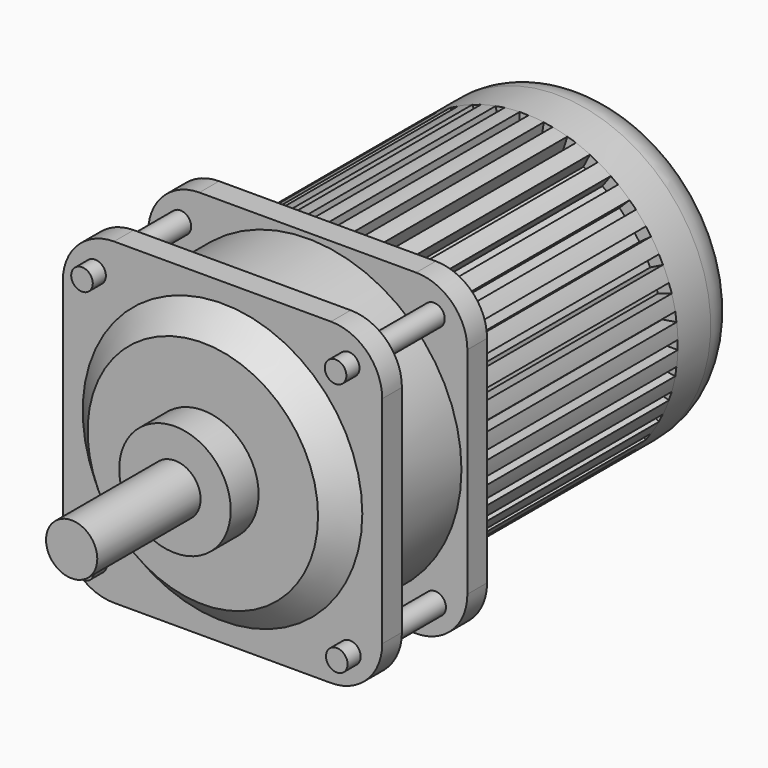
from build123d import *

# Parameters (mm, degrees)
F0_R           = 19.0502006096
F1_DEPTH       = 15.24
F1_DEPTH_BACK  = 15.24
F2_W           = 1.1123471195
F2_H           = 2.4813897908
F2_W_2         = 2.4813897908
F2_H_2         = 1.1123471195
F3_DEPTH       = 35.56
F4_R           = 19.0502006096
F5_DEPTH       = 10.16
F6_R           = 5.08
F8_DEPTH       = 3.048
F9_R           = 19.0452991295
F10_DEPTH      = 10.16
F12_DEPTH      = 3.048
F13_R          = 17.3253562596
F14_DEPTH      = 3.048
F15_SIZE       = 3.04799
F16_R          = 6.9123781537
F17_DEPTH      = 4.318
F18_R          = 3.1756298272
F19_DEPTH      = 16.002
F20_R          = 1.3365694891
F21_DEPTH      = 16.256
F21_DEPTH_BACK = 2.032


# Not quite as in the source:
# - a fillet or chamfer is up to 0.001 mm smaller than in the source, because OpenCascade refuses the exact size


with BuildPart() as f1:
    # F0 (on Front) → F1 (new body, two sides)
    with BuildSketch(Plane.XZ) as f1_sk:
        Circle(F0_R)
    extrude(amount=F1_DEPTH)
    extrude(f1_sk.sketch, amount=-F1_DEPTH_BACK)

    # F2 (on face) → F3 (cut)
    with BuildSketch(Plane.XZ.offset(15.24)):
        with Locations((0.0023364555, 18.4756238014)):
            Rectangle(F2_W, F2_H)
        Polygon((3.2477707136, 16.935368116), (3.6359455981, 19.3862078808), (2.5372933174, 19.5602173073), (2.149118433, 17.1093775425), align=None)
        Polygon((5.8570605182, 16.2188023577), (6.6238521332, 18.5787442876), (5.5659471569, 18.9224784512), (4.7991555418, 16.5625365212), align=None)
        Polygon((8.3221300544, 15.1028758582), (9.4486574456, 17.3138103508), (8.4575489049, 17.8188053755), (7.3310215138, 15.6078708829), align=None)
        Polygon((10.5822811291, 13.6150664315), (12.0408054533, 15.6225529419), (11.14089773, 16.2763741742), (9.6823734058, 14.2688876638), align=None)
        Polygon((12.5818613218, 11.7920088835), (14.3364688696, 13.5466164314), (13.5499206784, 14.3331646226), (11.7953131306, 12.5785570748), align=None)
        Polygon((14.271634332, 9.6785929414), (16.2791208424, 11.1371172656), (15.6252996101, 12.0370249889), (13.6178130997, 10.5785006647), align=None)
        Polygon((15.6099923401, 7.3268579196), (17.8209268327, 8.4533853107), (17.315931808, 9.4444938514), (15.1049973154, 8.3179664602), align=None)
        Polygon((16.5639805301, 4.7947113394), (18.9239224601, 5.5615029544), (18.5801882966, 6.6194079308), (16.2202463666, 5.8526163157), align=None)
        Polygon((17.1101085469, 2.1445030532), (19.5609483117, 2.5326779377), (19.3869388851, 3.6313302183), (16.9360991203, 3.2431553339), align=None)
        with Locations((18.4756238014, -0.0023364555)):
            Rectangle(F2_W_2, F2_H_2)
        Polygon((16.935368116, -3.2477707136), (19.3862078808, -3.6359455981), (19.5602173073, -2.5372933174), (17.1093775425, -2.149118433), align=None)
        Polygon((16.2188023577, -5.8570605182), (18.5787442876, -6.6238521332), (18.9224784512, -5.5659471569), (16.5625365212, -4.7991555418), align=None)
        Polygon((15.1028758582, -8.3221300544), (17.3138103508, -9.4486574456), (17.8188053755, -8.4575489049), (15.6078708829, -7.3310215138), align=None)
        Polygon((13.6150664315, -10.5822811291), (15.6225529419, -12.0408054533), (16.2763741742, -11.14089773), (14.2688876638, -9.6823734058), align=None)
        Polygon((11.7920088835, -12.5818613218), (13.5466164314, -14.3364688696), (14.3331646226, -13.5499206784), (12.5785570748, -11.7953131306), align=None)
        Polygon((9.6785929414, -14.271634332), (11.1371172656, -16.2791208424), (12.0370249889, -15.6252996101), (10.5785006647, -13.6178130997), align=None)
        Polygon((7.3268579196, -15.6099923401), (8.4533853107, -17.8209268327), (9.4444938514, -17.315931808), (8.3179664602, -15.1049973154), align=None)
        Polygon((4.7947113394, -16.5639805301), (5.5615029544, -18.9239224601), (6.6194079308, -18.5801882966), (5.8526163157, -16.2202463666), align=None)
        Polygon((2.1445030532, -17.1101085469), (2.5326779377, -19.5609483117), (3.6313302183, -19.3869388851), (3.2431553339, -16.9360991203), align=None)
        with Locations((-0.0023364555, -18.4756238014)):
            Rectangle(F2_W, F2_H)
        Polygon((-3.2477707136, -16.935368116), (-3.6359455981, -19.3862078808), (-2.5372933174, -19.5602173073), (-2.149118433, -17.1093775425), align=None)
        Polygon((-5.8570605182, -16.2188023577), (-6.6238521332, -18.5787442876), (-5.5659471569, -18.9224784512), (-4.7991555418, -16.5625365212), align=None)
        Polygon((-8.3221300544, -15.1028758582), (-9.4486574456, -17.3138103508), (-8.4575489049, -17.8188053755), (-7.3310215138, -15.6078708829), align=None)
        Polygon((-10.5822811291, -13.6150664315), (-12.0408054533, -15.6225529419), (-11.14089773, -16.2763741742), (-9.6823734058, -14.2688876638), align=None)
        Polygon((-12.5818613218, -11.7920088835), (-14.3364688696, -13.5466164314), (-13.5499206784, -14.3331646226), (-11.7953131306, -12.5785570748), align=None)
        Polygon((-14.271634332, -9.6785929414), (-16.2791208424, -11.1371172656), (-15.6252996101, -12.0370249889), (-13.6178130997, -10.5785006647), align=None)
        Polygon((-15.6099923401, -7.3268579196), (-17.8209268327, -8.4533853107), (-17.315931808, -9.4444938514), (-15.1049973154, -8.3179664602), align=None)
        Polygon((-16.5639805301, -4.7947113394), (-18.9239224601, -5.5615029544), (-18.5801882966, -6.6194079308), (-16.2202463666, -5.8526163157), align=None)
        Polygon((-17.1101085469, -2.1445030532), (-19.5609483117, -2.5326779377), (-19.3869388851, -3.6313302183), (-16.9360991203, -3.2431553339), align=None)
        with Locations((-18.4756238014, 0.0023364555)):
            Rectangle(F2_W_2, F2_H_2)
        Polygon((-16.935368116, 3.2477707136), (-19.3862078808, 3.6359455981), (-19.5602173073, 2.5372933174), (-17.1093775425, 2.149118433), align=None)
        Polygon((-16.2188023577, 5.8570605182), (-18.5787442876, 6.6238521332), (-18.9224784512, 5.5659471569), (-16.5625365212, 4.7991555418), align=None)
        Polygon((-15.1028758582, 8.3221300544), (-17.3138103508, 9.4486574456), (-17.8188053755, 8.4575489049), (-15.6078708829, 7.3310215138), align=None)
        Polygon((-13.6150664315, 10.5822811291), (-15.6225529419, 12.0408054533), (-16.2763741742, 11.14089773), (-14.2688876638, 9.6823734058), align=None)
        Polygon((-11.7920088835, 12.5818613218), (-13.5466164314, 14.3364688696), (-14.3331646226, 13.5499206784), (-12.5785570748, 11.7953131306), align=None)
        Polygon((-9.6785929414, 14.271634332), (-11.1371172656, 16.2791208424), (-12.0370249889, 15.6252996101), (-10.5785006647, 13.6178130997), align=None)
        Polygon((-7.3268579196, 15.6099923401), (-8.4533853107, 17.8209268327), (-9.4444938514, 17.315931808), (-8.3179664602, 15.1049973154), align=None)
        Polygon((-4.7947113394, 16.5639805301), (-5.5615029544, 18.9239224601), (-6.6194079308, 18.5801882966), (-5.8526163157, 16.2202463666), align=None)
        Polygon((-2.1445030532, 17.1101085469), (-2.5326779377, 19.5609483117), (-3.6313302183, 19.3869388851), (-3.2431553339, 16.9360991203), align=None)
    extrude(amount=-F3_DEPTH, mode=Mode.SUBTRACT)


with BuildPart() as f5:
    # F4 (on face) → F5 (new body)
    with BuildSketch(Plane(origin=(0, 15.24, 0), x_dir=(-1, 0, 0), z_dir=(0, 1, 0))):
        Circle(F4_R)
    extrude(amount=F5_DEPTH)

    # F6
    f6_edges = [f5.edges().sort_by_distance(p)[0] for p in [
        (19.050201, 25.4, 0),
    ]]
    fillet(f6_edges, radius=F6_R)


with BuildPart() as f8:
    # F7 (on face) → F8 (new body)
    with BuildSketch(Plane.XZ.offset(15.24)):
        with BuildLine():
            Line((-13.428560847, -19.6878351271), (13.428560847, -19.6878351271))
            ThreePointArc((13.428560847, -19.6878351271), (17.9186889076, -17.8279631876), (19.778560847, -13.3378351271))
            Line((19.778560847, -13.3378351271), (19.778560847, 13.3378351271))
            ThreePointArc((19.778560847, 13.3378351271), (17.9186889076, 17.8279631876), (13.428560847, 19.6878351271))
            Line((13.428560847, 19.6878351271), (-13.428560847, 19.6878351271))
            ThreePointArc((-13.428560847, 19.6878351271), (-17.9186889076, 17.8279631876), (-19.778560847, 13.3378351271))
            Line((-19.778560847, 13.3378351271), (-19.778560847, -13.3378351271))
            ThreePointArc((-19.778560847, -13.3378351271), (-17.9186889076, -17.8279631876), (-13.428560847, -19.6878351271))
        make_face()
    extrude(amount=F8_DEPTH)


with BuildPart() as f10:
    # F9 (on face) → F10 (new body)
    with BuildSketch(Plane.XZ.offset(18.288)):
        Circle(F9_R)
    extrude(amount=F10_DEPTH)


with BuildPart() as f12:
    # F11 (on face) → F12 (new body)
    with BuildSketch(Plane.XZ.offset(28.448)):
        with BuildLine():
            Line((-13.4440710932, -19.7128541768), (13.4440710932, -19.7128541768))
            ThreePointArc((13.4440710932, -19.7128541768), (17.9341991537, -17.8529822373), (19.7940710932, -13.3628541768))
            Line((19.7940710932, -13.3628541768), (19.7940710932, 13.3628541768))
            ThreePointArc((19.7940710932, 13.3628541768), (17.9341991537, 17.8529822373), (13.4440710932, 19.7128541768))
            Line((13.4440710932, 19.7128541768), (-13.4440710932, 19.7128541768))
            ThreePointArc((-13.4440710932, 19.7128541768), (-17.9341991537, 17.8529822373), (-19.7940710932, 13.3628541768))
            Line((-19.7940710932, 13.3628541768), (-19.7940710932, -13.3628541768))
            ThreePointArc((-19.7940710932, -13.3628541768), (-17.9341991537, -17.8529822373), (-13.4440710932, -19.7128541768))
        make_face()
    extrude(amount=F12_DEPTH)

    # F13 (on face) → F14 (join)
    with BuildSketch(Plane.XZ.offset(31.496)):
        Circle(F13_R)
    extrude(amount=F14_DEPTH)

    # F15 (size 3.048 in the source; OpenCascade refuses exactly that, so slightly less here)
    f15_edges = [f12.edges().sort_by_distance(p)[0] for p in [
        (-17.325356, -34.544, 0),
    ]]
    chamfer(f15_edges, length=F15_SIZE)

    # F16 (on face) → F17 (join)
    with BuildSketch(Plane.XZ.offset(34.544)):
        Circle(F16_R)
    extrude(amount=F17_DEPTH)


with BuildPart() as f19:
    # F18 (on face) → F19 (new body)
    with BuildSketch(Plane.XZ.offset(38.862)):
        Circle(F18_R)
    extrude(amount=F19_DEPTH)


with BuildPart() as f21:
    # F20 (on face) → F21 (new body, two sides)
    with BuildSketch(Plane.XZ.offset(31.496)) as f21_sk:
        with Locations((15.6389176846, 15.7868433744)):
            Circle(F20_R)
    extrude(amount=-F21_DEPTH)
    extrude(f21_sk.sketch, amount=F21_DEPTH_BACK)


with BuildPart() as f21b:
    # F20 (on face) → F21, piece 2 (new body, two sides)
    with BuildSketch(Plane.XZ.offset(31.496)) as f21_2_sk:
        with Locations((15.7868433744, -15.6389176846)):
            Circle(F20_R)
    extrude(amount=-F21_DEPTH)
    extrude(f21_2_sk.sketch, amount=F21_DEPTH_BACK)


with BuildPart() as f21c:
    # F20 (on face) → F21, piece 3 (new body, two sides)
    with BuildSketch(Plane.XZ.offset(31.496)) as f21_3_sk:
        with Locations((-15.6389176846, -15.7868433744)):
            Circle(F20_R)
    extrude(amount=-F21_DEPTH)
    extrude(f21_3_sk.sketch, amount=F21_DEPTH_BACK)


with BuildPart() as f21d:
    # F20 (on face) → F21, piece 4 (new body, two sides)
    with BuildSketch(Plane.XZ.offset(31.496)) as f21_4_sk:
        with Locations((-15.7868433744, 15.6389176846)):
            Circle(F20_R)
    extrude(amount=-F21_DEPTH)
    extrude(f21_4_sk.sketch, amount=F21_DEPTH_BACK)


solid = Compound([f1.part, f5.part, f8.part, f10.part, f12.part, f19.part, f21.part, f21b.part, f21c.part, f21d.part])
